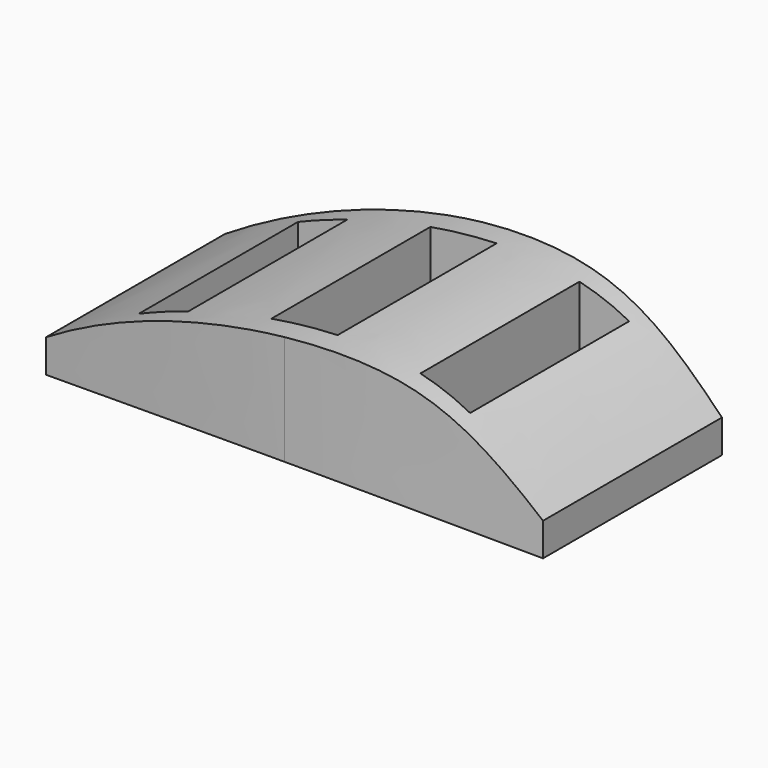
from build123d import *

# Parameters (mm, degrees)
F5_DEPTH  = 38.1
F8_DEPTH  = 30.734
F9_W      = 7.62
F9_H      = 15.24
F9_W_2    = 10.16
F10_DEPTH = 25.4


# Not quite as in the source:
# - a feature of the source that left no trace in its solid (it failed there, or was rolled back) is left out


with BuildPart() as f5:
    # F3 (on face) → F5 (new body)
    with BuildSketch(Plane.XZ.offset(38.1)):
        with BuildLine():
            Line((0, 5.08), (0, 0))
            add(Edge.make_bspline(
                [(0, 0), (12.7, 0.707683037), (38.1, 2.1230491111), (63.5, 0.707683037), (76.2, 0)],
                knots=[0, 0, 0, 0, 0.5, 1, 1, 1, 1], degree=3))
            Line((76.2, 0), (76.2, 5.08))
            add(Edge.make_bspline(
                [(0, 5.08), (17.1016856021, 15.7050435078), (52.4364024312, 22.8591352455), (67.3437483547, 13.2911519776), (76.2, 5.08)],
                knots=[0, 0, 0, 0, 0.5766084835, 1, 1, 1, 1], degree=3))
        make_face()
    extrude(amount=-F5_DEPTH)

    # F7 (on offset) → F8 (cut)
    with BuildSketch(Plane.XY.offset(25.4)):
        with BuildLine():
            Line((0, -38.1), (38.1, -38.1))
            add(Edge.make_bspline(
                [(0, -36.195), (12.7, -37.1475), (25.4, -38.1), (38.1, -38.1)],
                knots=[0, 0, 0, 0, 0.5, 0.5, 0.5, 0.5], degree=3))
            Line((0, -36.195), (0, -38.1))
        make_face()
        with BuildLine():
            add(Edge.make_bspline(
                [(38.1, -38.1), (50.8, -38.1), (63.5, -37.1475), (76.2, -36.195)],
                knots=[0.5, 0.5, 0.5, 0.5, 1, 1, 1, 1], degree=3))
            Line((38.1, -38.1), (76.2, -38.1))
            Line((76.2, -38.1), (76.2, -36.195))
        make_face()
        with BuildLine():
            Line((76.2, 0), (38.1, 0))
            add(Edge.make_bspline(
                [(38.1, 0), (50.8, 0), (63.5, -0.9525), (76.2, -1.905)],
                knots=[0.5, 0.5, 0.5, 0.5, 1, 1, 1, 1], degree=3))
            Line((76.2, -1.905), (76.2, 0))
        make_face()
        with BuildLine():
            Line((38.1, 0), (0, 0))
            Line((0, 0), (0, -1.905))
            add(Edge.make_bspline(
                [(0, -1.905), (12.7, -0.9525), (25.4, 0), (38.1, 0)],
                knots=[0, 0, 0, 0, 0.5, 0.5, 0.5, 0.5], degree=3))
        make_face()
    extrude(amount=-F8_DEPTH, mode=Mode.SUBTRACT)

    # F9 (on offset) → F10 (cut)
    with BuildSketch(Plane.XY.offset(25.4)):
        with Locations((59.69, -11.43)):
            Rectangle(F9_W, F9_H)
        with Locations((59.69, -26.67)):
            Rectangle(F9_W, F9_H)
        with Locations((38.1, -26.67)):
            Rectangle(F9_W_2, F9_H)
        with Locations((38.1, -11.43)):
            Rectangle(F9_W_2, F9_H)
        with Locations((16.51, -26.67)):
            Rectangle(F9_W, F9_H)
        with Locations((16.51, -11.43)):
            Rectangle(F9_W, F9_H)
    extrude(amount=-F10_DEPTH, mode=Mode.SUBTRACT)


solid = f5.part
